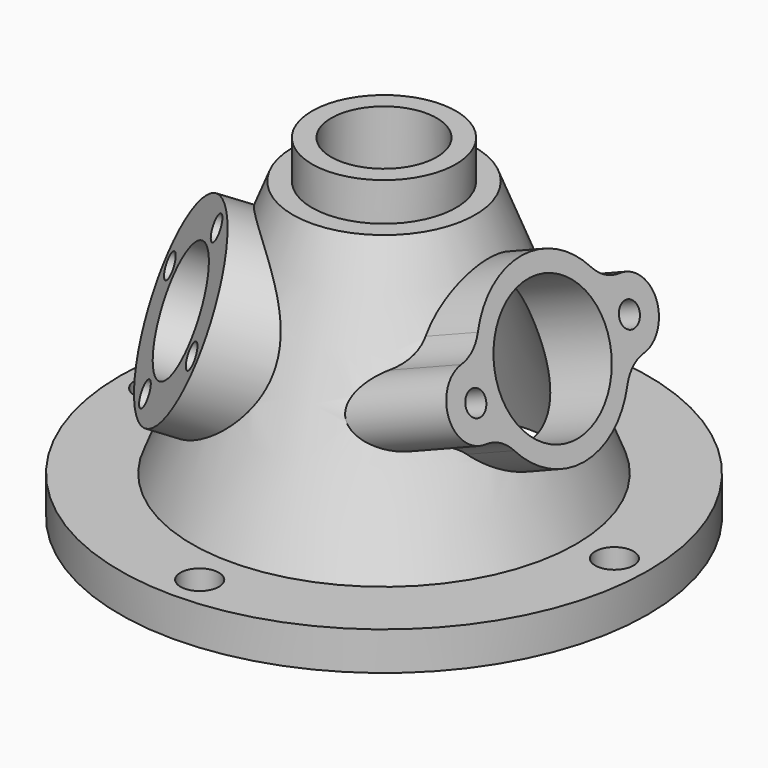
from build123d import *

# Parameters (mm, degrees)
F8_D      = 14
F8_DEPTH  = 11
F8_TIP    = 4.2060243332
F9_D      = 2.5
F9_DEPTH  = 11
F9_TIP    = 0.7510757738
F13_R     = 10
F15_D     = 12
F15_DEPTH = 10
F15_TIP   = 3.6051637142
F16_D     = 2.5
F16_DEPTH = 10
F16_TIP   = 0.7510757738
F18_D     = 4
F18_DEPTH = 4
F18_TIP   = 1.2017212381
F19_SCALE = 5


with BuildPart() as f1:
    # F0 (on Front) → F1 (revolve)
    with BuildSketch(Plane.XZ):
        Polygon((-27.5, 4), (-27.5, 0), (-19.4194839306, 0), (-8.1356925013, 28.7928420941), (-5.5, 28.7928420941), (-5.5, 34.7928420941), (-7.5, 34.7928420941), (-7.5, 30.7928420941), (-9.5, 30.7928420941), (-20, 4), align=None)
    revolve(axis=Axis((0, 0, 21.2173005566), (0, 0, -1)))

    # F5 (on offset) → F6 (join, up to the next surface of F1)
    with BuildSketch(Plane(origin=(22.0989238728, 0, 8.7049976133), x_dir=(0, -1, 0), z_dir=(-0.930417568, 0, -0.3665012267))):
        with BuildLine():
            ThreePointArc((10.2975, 15.8592048537), (8.6439141314, 16.3769317522), (7.3644230769, 17.545388002))
            ThreePointArc((7.3644230769, 17.545388002), (0, 21.3718715244), (-7.3644230769, 17.545388002))
            ThreePointArc((-7.3644230769, 17.545388002), (-8.6439141314, 16.3769317522), (-10.2975, 15.8592048537))
            ThreePointArc((-10.2975, 15.8592048537), (-13.5, 12.3718715244), (-10.2975, 8.884538195))
            ThreePointArc((-10.2975, 8.884538195), (-8.6439141314, 8.3668112965), (-7.3644230769, 7.1983550468))
            ThreePointArc((-7.3644230769, 7.1983550468), (0, 3.3718715244), (7.3644230769, 7.1983550468))
            ThreePointArc((7.3644230769, 7.1983550468), (8.6439141314, 8.3668112965), (10.2975, 8.884538195))
            ThreePointArc((10.2975, 8.884538195), (13.5, 12.3718715244), (10.2975, 15.8592048537))
        make_face()
    extrude(until=Until.NEXT)

    # F8
    with Locations(Plane(origin=(22.0989238728, 0, 8.7049976133), x_dir=(0, 1, 0), z_dir=(0.930417568, 0, 0.3665012267))):
        with Locations((0, 12.3718715244)):
            Hole(F8_D / 2, depth=F8_DEPTH)
            with Locations((0, 0, -(F8_DEPTH + F8_TIP / 2))):  # 118° drill point
                Cone(0, F8_D / 2, F8_TIP, mode=Mode.SUBTRACT)

    # F9
    with Locations(Plane(origin=(22.0989238728, 0, 8.7049976133), x_dir=(0, 1, 0), z_dir=(0.930417568, 0, 0.3665012267))):
        with Locations((-10, 12.3718715244), (10, 12.3718715244)):
            Hole(F9_D / 2, depth=F9_DEPTH)
            with Locations((0, 0, -(F9_DEPTH + F9_TIP / 2))):  # 118° drill point
                Cone(0, F9_D / 2, F9_TIP, mode=Mode.SUBTRACT)

    # F13 (on face) → F14 (join, up to the next surface of F1)
    with BuildSketch(Plane(origin=(-14.9683943558, -14.9683943558, 8.3384963866), x_dir=(-0.7531013043, 0.5747413036, -0.3201731708), z_dir=(0.6579045717, 0.6579045717, -0.3665012267))):
        with Locations((-4.2573802039, 11.6162781826)):
            Circle(F13_R)
    extrude(until=Until.NEXT)

    # F15
    with Locations(Plane(origin=(-14.9683943558, -14.9683943558, 8.3384963866), x_dir=(-0.7531013043, 0.5747413036, -0.3201731708), z_dir=(-0.6579045717, -0.6579045717, 0.3665012267))):
        with Locations((-4.2573802039, -11.6162781826)):
            Hole(F15_D / 2, depth=F15_DEPTH)
            with Locations((0, 0, -(F15_DEPTH + F15_TIP / 2))):  # 118° drill point
                Cone(0, F15_D / 2, F15_TIP, mode=Mode.SUBTRACT)

    # F16
    with Locations(Plane(origin=(-14.9683943558, -14.9683943558, 8.3384963866), x_dir=(-0.7531013043, 0.5747413036, -0.3201731708), z_dir=(-0.6579045717, -0.6579045717, 0.3665012267))):
        with Locations((-7.0103219528, -19.127690282), (3.2540318955, -14.3692199314), (-1.504438455, -4.1048660832), (-11.7687923033, -8.8633364337)):
            Hole(F16_D / 2, depth=F16_DEPTH)
            with Locations((0, 0, -(F16_DEPTH + F16_TIP / 2))):  # 118° drill point
                Cone(0, F16_D / 2, F16_TIP, mode=Mode.SUBTRACT)

    # F18
    with Locations(Plane(origin=(0, 0, 0), x_dir=(1, 0, 0), z_dir=(0, 0, -1))):
        with Locations((-24, 0), (0, 24), (24, 0), (0, -24)):
            Hole(F18_D / 2, depth=F18_DEPTH)
            with Locations((0, 0, -(F18_DEPTH + F18_TIP / 2))):  # 118° drill point
                Cone(0, F18_D / 2, F18_TIP, mode=Mode.SUBTRACT)


with BuildPart() as f1_1:
    # F19: moved
    add(f1.part.scale(F19_SCALE))


solid = f1_1.part
